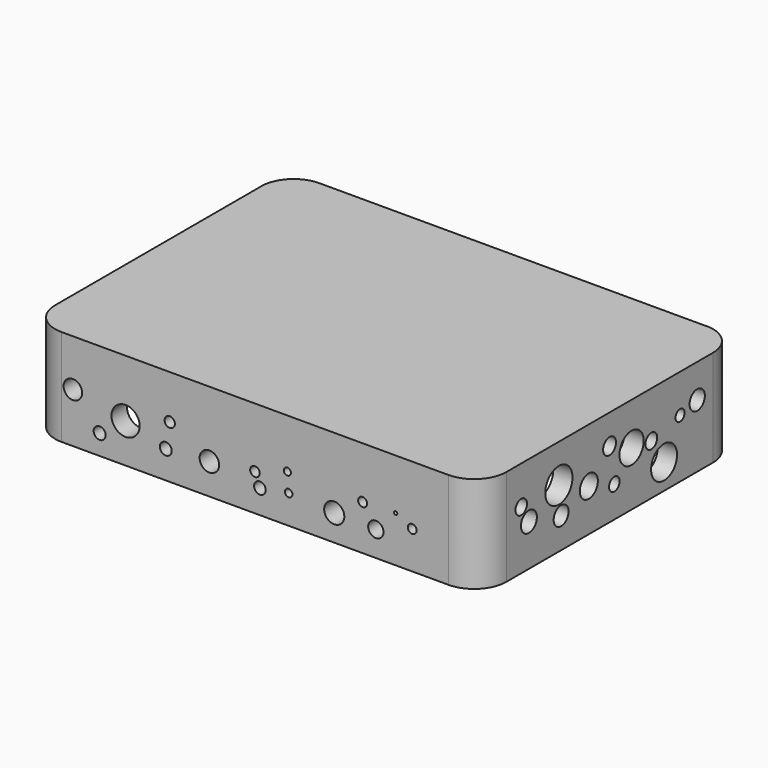
from build123d import *

# Parameters (mm, degrees)
F1_DEPTH  = 38.1
F6_T      = -7.62
F7_DEPTH  = 38.1
F10_R     = 3.4402348101
F10_R_2   = 1.4505288856
F10_R_3   = 3.2596601753
F10_R_4   = 1.3950746304
F10_R_5   = 2.2588254498
F10_R_6   = 1.8383712519
F10_R_7   = 1.4907687616
F10_R_8   = 1.2973945839
F10_R_9   = 1.83837131
F10_R_10  = 1.0320693254
F10_R_11  = 3.8119505804
F10_R_12  = 4.1679066842
F10_R_13  = 1.1524641388
F10_R_14  = 3.3393658282
F11_DEPTH = 25.4
F12_R     = 3.6570226398
F12_R_2   = 2.3640747981
F12_R_3   = 5.5483952241
F12_R_4   = 2.0326172526
F12_R_5   = 2.3458634607
F12_R_6   = 3.8447490406
F12_R_7   = 1.8933108358
F12_R_8   = 1.4014887984
F12_R_9   = 1.472197321
F12_R_10  = 2.3058218012
F12_R_11  = 1.7698934625
F12_R_12  = 0.6506260484
F12_R_13  = 1.7458093881
F12_R_14  = 3.0182277356
F12_R_15  = 3.9725453558
F13_DEPTH = 7.874
F14_R     = 2.8349830175
F14_R_2   = 5.493985489
F14_R_3   = 2.9616527697
F14_R_4   = 3.5302276567
F14_R_5   = 4.8656757899
F14_R_6   = 2.9850116345
F14_R_7   = 1.2599919894
F14_R_8   = 2.3233110537
F14_R_9   = 3.8321169211
F14_R_10  = 2.1503087946
F14_R_11  = 1.5237568978
F15_DEPTH = 25.4
F16_R     = 2.8430027376
F16_R_2   = 6.7189755212
F16_R_3   = 3.9338718219
F16_R_4   = 3.6647015935
F16_R_5   = 2.5889575184
F16_R_6   = 2.894541857
F16_R_7   = 2.2200135957
F16_R_8   = 3.7674866617
F16_R_9   = 6.390010833
F16_R_10  = 3.1763387686
F16_R_11  = 4.4400246889
F16_R_12  = 5.9672503681
F17_DEPTH = 7.62


# Not quite as in the source:
# - a feature names something its author has since deleted; it is built from what else it names


with BuildPart() as f1:
    # F0 (on Top) → F1 (new body)
    with BuildSketch(Plane.XY):
        with BuildLine():
            Line((-76.2, -63.5), (76.2, -63.5))
            ThreePointArc((76.2, -63.5), (85.1802561211, -59.7802561211), (88.9, -50.8))
            Line((88.9, -50.8), (88.9, 50.8837117171))
            ThreePointArc((88.9, 50.8837117171), (84.6499025139, 60.364700458), (74.7442287394, 63.5))
            Line((74.7442287394, 63.5), (-31.496, 63.5))
            Line((-31.496, 63.5), (-51.816, 63.5))
            Line((-51.816, 63.5), (-76.2, 63.5))
            ThreePointArc((-76.2, 63.5), (-85.1802561211, 59.7802561211), (-88.9, 50.8))
            Line((-88.9, 50.8), (-88.9, -50.8))
            ThreePointArc((-88.9, -50.8), (-85.1802561211, -59.7802561211), (-76.2, -63.5))
        make_face()
        with BuildLine():
            ThreePointArc((64.5057426338, -17.1976926005), (29.972759331, -52.6140458587), (-4.5602239718, -17.1976926005))
            ThreePointArc((-4.5602239718, -17.1976926005), (29.972759331, 16.4739541413), (64.5057426338, -17.1976926005))
        make_face(mode=Mode.SUBTRACT)
        with BuildLine():
            ThreePointArc((64.5057426338, -17.1976926005), (29.972759331, 16.4739541413), (-4.5602239718, -17.1976926005))
            Line((-4.5602239718, -17.1976926005), (64.5057426338, -17.1976926005))
        make_face()
        with BuildLine():
            Line((64.5057426338, -17.1976926005), (-4.5602239718, -17.1976926005))
            ThreePointArc((-4.5602239718, -17.1976926005), (29.972759331, -52.6140458587), (64.5057426338, -17.1976926005))
        make_face()
    extrude(amount=F1_DEPTH)

    # F6
    f6_openings = [f1.faces().sort_by_distance(p)[0] for p in [
        (0.004184, 0.003111, 0),
    ]]
    offset(amount=F6_T, openings=f6_openings, kind=Kind.INTERSECTION)

    # F0 (on Top) → F7 (join)
    with BuildSketch(Plane.XY):
        with BuildLine():
            Line((64.5057426338, -17.1976926005), (-4.5602239718, -17.1976926005))
            ThreePointArc((-4.5602239718, -17.1976926005), (29.972759331, -52.6140458587), (64.5057426338, -17.1976926005))
        make_face()
        with BuildLine():
            ThreePointArc((64.5057426338, -17.1976926005), (29.972759331, 16.4739541413), (-4.5602239718, -17.1976926005))
            Line((-4.5602239718, -17.1976926005), (64.5057426338, -17.1976926005))
        make_face()
    extrude(amount=F7_DEPTH)

    # F8 (on face) → F9 (revolve, cut)
    with BuildSketch(Plane.XY):
        with BuildLine():
            Line((64.328390356, -18.9051141856), (-4.4528775117, -17.6680727243))
            ThreePointArc((-4.4528775117, -17.6680727243), (29.3206857453, -52.5966023324), (64.328390356, -18.9051141856))
        make_face()
    revolve(axis=Axis((29.9377564222, -18.2865934549, 0), (0.9998383064, -0.0179822425, 0)), mode=Mode.SUBTRACT)

    # F10 (on face) → F11 (cut)
    with BuildSketch(Plane(origin=(0, 63.5, 0), x_dir=(-1, 0, 0), z_dir=(0, 1, 0))):
        with Locations((-61.6375170648, 26.3894759119)):
            Circle(F10_R)
        with Locations((-47.8765815496, 10.6790764257)):
            Circle(F10_R_2)
        with Locations((-27.6938788593, 19.1649850458)):
            Circle(F10_R_3)
        with Locations((8.0845486373, 18.9356375486)):
            Circle(F10_R_4)
        with Locations((13.3595727384, 10.9084257856)):
            Circle(F10_R_5)
        with Locations((-7.5111761689, 7.9268896952)):
            Circle(F10_R_6)
        with Locations((24.5976690203, 22.2611948848)):
            Circle(F10_R_7)
        with Locations((39.275996387, 27.880243957)):
            Circle(F10_R_8)
        with Locations((39.5053476095, 18.247589469)):
            Circle(F10_R_9)
        with Locations((41.6841618717, 6.5507958643)):
            Circle(F10_R_10)
        with Locations((-64.389705658, 5.7480754331)):
            Circle(F10_R_11)
        with Locations((66.4538443089, 13.2019137964)):
            Circle(F10_R_12)
        with Locations((74.7103989124, 35.4487560689)):
            Circle(F10_R_13)
        with Locations((70.0087472796, 4.027958028)):
            Circle(F10_R_14)
    extrude(amount=-F11_DEPTH, mode=Mode.SUBTRACT)

    # F12 (on face) → F13 (cut)
    with BuildSketch(Plane.XZ.offset(63.5)):
        with Locations((-71.7288702726, 19.6236837655)):
            Circle(F12_R)
        with Locations((-61.1788183451, 7.9268896952)):
            Circle(F12_R_2)
        with Locations((-50.9727932513, 15.4954027385)):
            Circle(F12_R_3)
        with Locations((-33.5708744824, 20.7350011915)):
            Circle(F12_R_4)
        with Locations((-35.1323746145, 10.975622572)):
            Circle(F12_R_5)
        with Locations((-17.955865711, 12.1467476711)):
            Circle(F12_R_6)
        with Locations((0, 14.4889988005)):
            Circle(F12_R_7)
        with Locations((12.7536486834, 18.6530016363)):
            Circle(F12_R_8)
        with Locations((13.2741490379, 11.365997605)):
            Circle(F12_R_9)
        with Locations((1.9532681908, 9.4141215086)):
            Circle(F12_R_10)
        with Locations((42.4221642315, 17.7421253175)):
            Circle(F12_R_11)
        with Locations((55.4346702993, 18.1325003505)):
            Circle(F12_R_12)
        with Locations((61.9409233332, 14.7492494434)):
            Circle(F12_R_13)
        with Locations((47.6271659136, 9.9346218631)):
            Circle(F12_R_14)
        with Locations((31.2314070761, 10.3249968961)):
            Circle(F12_R_15)
    extrude(amount=-F13_DEPTH, mode=Mode.SUBTRACT)

    # F14 (on face) → F15 (cut)
    with BuildSketch(Plane(origin=(-88.9, 0, 0), x_dir=(0, -1, 0), z_dir=(-1, 0, 0))):
        with Locations((-41.8995916843, 20.8350885659)):
            Circle(F14_R)
        with Locations((-19.0784204751, 17.0315597206)):
            Circle(F14_R_2)
        with Locations((11.7724230513, 21.3985741138)):
            Circle(F14_R_3)
        with Locations((27.5500230491, 17.4541734159)):
            Circle(F14_R_4)
        with Locations((44.4545932114, 18.862888217)):
            Circle(F14_R_5)
        with Locations((29.9448370934, 25.0612311065)):
            Circle(F14_R_6)
        with Locations((13.6037515476, 9.2836311087)):
            Circle(F14_R_7)
        with Locations((1.4888086589, 5.90271689)):
            Circle(F14_R_8)
        with Locations((-6.2591200694, 16.890687868)):
            Circle(F14_R_9)
        with Locations((-29.9255196005, 9.0018883348)):
            Circle(F14_R_10)
        with Locations((-44.1535338759, 6.1844596639)):
            Circle(F14_R_11)
    extrude(amount=-F15_DEPTH, mode=Mode.SUBTRACT)

    # F16 (on face) → F17 (cut)
    with BuildSketch(Plane.YZ.offset(88.9)):
        with Locations((-43.4940196574, 22.9858383536)):
            Circle(F16_R)
        with Locations((-24.9705445021, 22.9858383536)):
            Circle(F16_R_2)
        with Locations((-39.7265329957, 16.392737627)):
            Circle(F16_R_3)
        with Locations((-23.8716956228, 11.9973365217)):
            Circle(F16_R_4)
        with Locations((2.3437284399, 12.3112937436)):
            Circle(F16_R_5)
        with Locations((20.5532442778, 19.8462661356)):
            Circle(F16_R_6)
        with Locations((34.6813164651, 22.9858383536)):
            Circle(F16_R_7)
        with Locations((43.1581586599, 24.8695798218)):
            Circle(F16_R_8)
        with Locations((26.8323868513, 9.9566150457)):
            Circle(F16_R_9)
        with Locations((0, 26.4393668622)):
            Circle(F16_R_10)
        with Locations((-10.2145588025, 16.7066939175)):
            Circle(F16_R_11)
        with Locations((10.8205722645, 21.4160531759)):
            Circle(F16_R_12)
    extrude(amount=-F17_DEPTH, mode=Mode.SUBTRACT)


solid = f1.part
